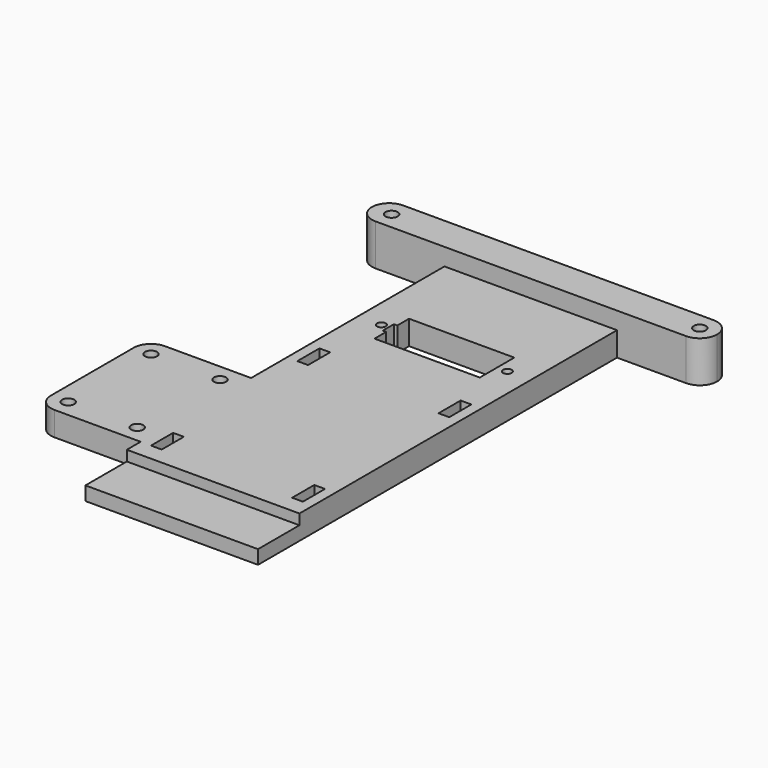
from build123d import *

# Parameters (mm, degrees)
F0_W     = 3.1029209495
F0_H     = 8
F0_R     = 1.25
F1_DEPTH = 7
F0_R_2   = 1.75
F2_DEPTH = 12
F0_W_2   = 30
F0_H_2   = 40
F3_DEPTH = 7
F4_R     = 5
F5_R     = 1.75
F6_DEPTH = 25
F0_W_3   = 50
F0_H_3   = 15
F7_DEPTH = 4


with BuildPart() as f1:
    # F0 (on Top) → F1 (new body)
    with BuildSketch(Plane.XY):
        Polygon((25, -50), (25, 65), (-25, 65), (-25, -5), (-25, -45), (-25, -50), align=None)
        with Locations((-20.4485395253, -41)):
            Rectangle(F0_W, F0_H, mode=Mode.SUBTRACT)
        with Locations((20.4485395253, -41)):
            Rectangle(F0_W, F0_H, mode=Mode.SUBTRACT)
        with Locations((-20.4485395253, 12)):
            Rectangle(F0_W, F0_H, mode=Mode.SUBTRACT)
        with Locations((-18.25, 33.75)):
            Circle(F0_R, mode=Mode.SUBTRACT)
        with Locations((20.4485395253, 12)):
            Rectangle(F0_W, F0_H, mode=Mode.SUBTRACT)
        Polygon((15.25, 40), (15.25, 27.5), (-15.25, 27.5), (-15.25, 31.75), (-16.25, 31.75), (-16.25, 35.75), (-15.25, 35.75), (-15.25, 40), align=None, mode=Mode.SUBTRACT)
        with Locations((18.25, 33.75)):
            Circle(F0_R, mode=Mode.SUBTRACT)
    extrude(amount=F1_DEPTH)

    # F0 (on Top) → F2 (join)
    with BuildSketch(Plane.XY):
        with BuildLine():
            Line((-25, 65), (25, 65))
            Line((25, 65), (45, 65))
            ThreePointArc((45, 65), (48.5355339059, 66.4644660941), (50, 70))
            ThreePointArc((50, 70), (48.5355339059, 73.5355339059), (45, 75))
            Line((45, 75), (-45, 75))
            ThreePointArc((-45, 75), (-48.5355339059, 73.5355339059), (-50, 70))
            ThreePointArc((-50, 70), (-48.5355339059, 66.4644660941), (-45, 65))
            Line((-45, 65), (-25, 65))
        make_face()
        with Locations((-44.2887660861, 70)):
            Circle(F0_R_2, mode=Mode.SUBTRACT)
        with Locations((45, 70)):
            Circle(F0_R_2, mode=Mode.SUBTRACT)
    extrude(amount=F2_DEPTH)

    # F0 (on Top) → F3 (join)
    with BuildSketch(Plane.XY):
        with Locations((-40, -25)):
            Rectangle(F0_W_2, F0_H_2)
    extrude(amount=F3_DEPTH)

    # F4
    f4_edges = [f1.edges().sort_by_distance(p)[0] for p in [
        (-55, -5, 3.5),
        (-55, -45, 3.5),
    ]]
    fillet(f4_edges, radius=F4_R)

    # F5 (on face) → F6 (cut)
    with BuildSketch(Plane.XY.offset(7)):
        with Locations((-50, -10)):
            Circle(F5_R)
        with Locations((-30, -10)):
            Circle(F5_R)
        with Locations((-30, -40)):
            Circle(F5_R)
        with Locations((-50, -40)):
            Circle(F5_R)
    extrude(amount=-F6_DEPTH, mode=Mode.SUBTRACT)

    # F0 (on Top) → F7 (join)
    with BuildSketch(Plane.XY):
        with Locations((0, -57.5)):
            Rectangle(F0_W_3, F0_H_3)
    extrude(amount=F7_DEPTH)


solid = f1.part
